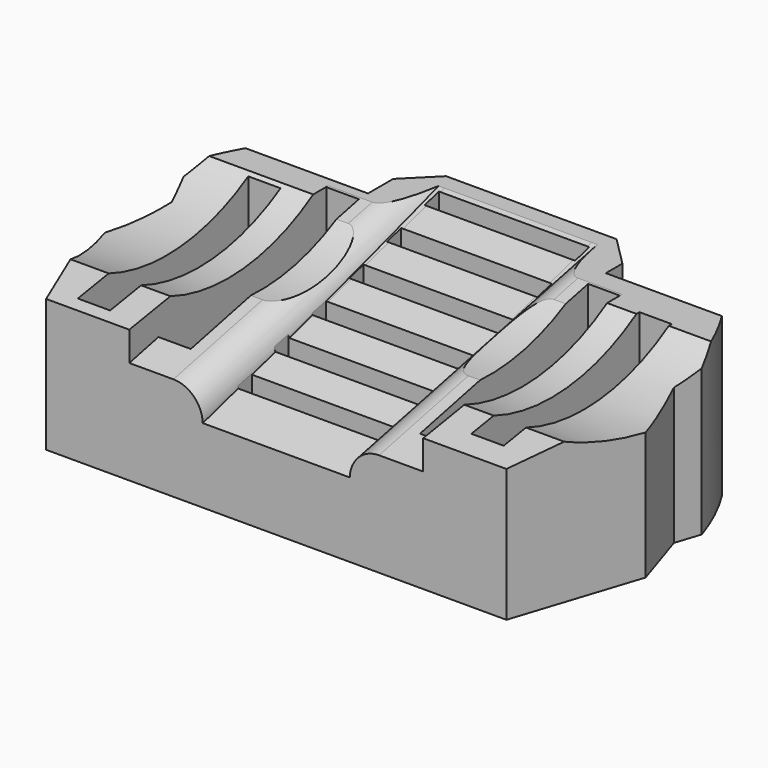
from build123d import *

# Parameters (mm, degrees)
F1_START       = 19.05
F1_DEPTH       = 31.75
F3_DEPTH       = 12.7
F5_DEPTH       = 25.4
F7_DEPTH       = 50.8
F10_T4_DEPTH   = 118.8107467306
F10_T9_DEPTH   = 118.8107467306
F11_W          = 5.588
F11_H          = 36.83
F11_H_2        = 36.322
F12_DEPTH      = 25.4
F12_DEPTH_BACK = 19.05
F13_W          = 26.0096
F13_H          = 3.048
F14_DEPTH      = 19.05
F15_W          = 26.0096
F15_H          = 3.048
F15_W_2        = 25.684906454
F16_DEPTH      = 25.4
F17_R          = 34.3708732133
F18_DEPTH      = 63.5
F19_W          = 101.6
F19_H          = 32.0445634425
F19_W_2        = 28.5529913381
F19_H_2        = 6.6054575145
F19_H_3        = 10.527446866
F19_W_3        = 20.7230086619
F19_H_4        = 8.6696632206
F19_H_5        = 7.8439861536
F20_DEPTH      = 38.1
F21_SIZE       = 5.08


# Not quite as in the source:
# - a fillet or chamfer that OpenCascade refuses, or shapes differently, is made with other operations: its cross-section is extruded or revolved along the edge and cut away or added
# - a feature of the source that left no trace in its solid (it failed there, or was rolled back) is left out


with BuildPart() as f1:
    # F0 (on Top) → F1 (new body)
    with BuildSketch(Plane.XY.offset(F1_START)):
        Polygon((-27.681270317, -38.1), (-23.1827056925, -38.1), (-29.0714032363, -33.8216107999), align=None)
        Polygon((-29.0714032363, -33.8216107999), (-23.1827056925, -38.1), (23.1827056925, -38.1), (29.0714032363, -33.8216107999), (43.3991033054, 10.2745158286), (41.1498209932, 17.1970949714), (3.6394152315, 44.45), (-3.6394152315, 44.45), (-41.1498209932, 17.1970949714), (-43.3991033054, 10.2745158286), align=None)
        with BuildLine():
            Line((23.1827056925, -38.1), (-23.1827056925, -38.1))
            Line((-23.1827056925, -38.1), (-27.681270317, -38.1))
            ThreePointArc((-27.681270317, -38.1), (0, -47.0941899427), (27.681270317, -38.1))
            Line((27.681270317, -38.1), (23.1827056925, -38.1))
        make_face()
        Polygon((-37.8114284312, -27.4716107999), (-29.0714032363, -33.8216107999), (-43.3991033054, 10.2745158286), (-46.7374958674, 0), align=None)
        Polygon((29.0714032363, -33.8216107999), (23.1827056925, -38.1), (27.681270317, -38.1), align=None)
        Polygon((-44.7892362247, 14.5529050286), (-43.3991033054, 10.2745158286), (-41.1498209932, 17.1970949714), align=None)
        Polygon((43.3991033054, 10.2745158286), (29.0714032363, -33.8216107999), (37.8114284312, -27.4716107999), (46.7374958674, 0), align=None)
        with BuildLine():
            Line((-44.7892362247, 14.5529050286), (-41.1498209932, 17.1970949714))
            Line((-41.1498209932, 17.1970949714), (-3.6394152315, 44.45))
            Line((-3.6394152315, 44.45), (0, 47.0941899427))
            ThreePointArc((0, 47.0941899427), (-27.681270317, 38.1), (-44.7892362247, 14.5529050286))
        make_face()
        Polygon((41.1498209932, 17.1970949714), (43.3991033054, 10.2745158286), (44.7892362247, 14.5529050286), align=None)
        Polygon((0, 47.0941899427), (-3.6394152315, 44.45), (3.6394152315, 44.45), align=None)
        with BuildLine():
            ThreePointArc((44.7892362247, 14.5529050286), (27.681270317, 38.1), (0, 47.0941899427))
            Line((0, 47.0941899427), (3.6394152315, 44.45))
            Line((3.6394152315, 44.45), (41.1498209932, 17.1970949714))
            Line((41.1498209932, 17.1970949714), (44.7892362247, 14.5529050286))
        make_face()
    extrude(amount=F1_DEPTH)

    # F2 (on Right) → F3 (cut, symmetric)
    with BuildSketch(Plane.YZ):
        Polygon((-44.8449260175, 25.4), (69.4550739825, 57.15), (-44.8449260175, 57.15), align=None)
    extrude(amount=F3_DEPTH, both=True, mode=Mode.SUBTRACT)

    # F4 (on Right) → F5 (cut, symmetric)
    with BuildSketch(Plane.YZ):
        Polygon((-44.8449260175, 31.75), (70.0721293688, 57.15), (-44.8449260175, 57.15), align=None)
    extrude(amount=F5_DEPTH, both=True, mode=Mode.SUBTRACT)

    # F6 (on Right) → F7 (cut, symmetric)
    with BuildSketch(Plane.YZ):
        Polygon((69.4550739825, 57.15), (-44.8449260175, 57.15), (-44.8449260175, 38.1), (5.1235620631, 46.4280813468), (48.464309937, 53.6515393258), align=None)
        Polygon((48.464309937, 46.4280813468), (48.464309937, 53.6515393258), (5.1235620631, 46.4280813468), align=None)
    extrude(amount=F7_DEPTH, both=True, mode=Mode.SUBTRACT)

    # F10: fillet of radius 5.08 on 2 edges, made by hand


with BuildPart() as f10_tool2:
    # F10_s3 → F10_t4 (new body)
    with BuildSketch(Plane(origin=(0, -48.4660281995, -10.712396973), x_dir=(1, 0, 0), z_dir=(0, 0.9764331595, 0.2158200292))):
        with BuildLine():
            ThreePointArc((-12.7, -35.6001860579), (-14.1878975516, -39.1922885063), (-17.78, -40.6801860579))
            Line((-17.78, -40.6801860579), (-12.7, -40.6801860579))
            Line((-12.7, -40.6801860579), (-12.7, -35.6001860579))
        make_face()
    extrude(amount=F10_T4_DEPTH)

    split(bisect_by=Plane(origin=(0, -9.762530517, 35.1451098613), x_dir=(1, 0, 0), z_dir=(0, -0.2676438638, 0.9635179096)), keep=Keep.TOP)


with BuildPart() as f1_1:
    add(f1.part)

    # F10_t1: cut F10_tool2
    add(f10_tool2.part, mode=Mode.SUBTRACT)


with BuildPart() as f10_tool7:
    # F10_s8 → F10_t9 (new body)
    with BuildSketch(Plane(origin=(0, -48.4660281995, -10.712396973), x_dir=(1, 0, 0), z_dir=(0, 0.9764331595, 0.2158200292))):
        with BuildLine():
            ThreePointArc((17.78, -40.6801860579), (14.1878975516, -39.1922885063), (12.7, -35.6001860579))
            Line((12.7, -35.6001860579), (12.7, -40.6801860579))
            Line((12.7, -40.6801860579), (17.78, -40.6801860579))
        make_face()
    extrude(amount=F10_T9_DEPTH)

    split(bisect_by=Plane(origin=(0, -9.762530517, 35.1451098613), x_dir=(1, 0, 0), z_dir=(0, -0.2676438638, 0.9635179096)), keep=Keep.TOP)


with BuildPart() as f1_2:
    add(f1_1.part)

    # F10_t6: cut F10_tool7
    add(f10_tool7.part, mode=Mode.SUBTRACT)

    # F11 (on offset) → F12 (cut, two sides)
    with BuildSketch(Plane.XY.offset(50.8)) as f12_sk:
        with Locations((-33.274, -0.7722239547)):
            Rectangle(F11_W, F11_H)
        with Locations((-22.606, 3.0599313468)):
            Rectangle(F11_W, F11_H_2)
        with Locations((33.274, 0.82358277)):
            Rectangle(F11_W, F11_H_2)
        with Locations((22.606, 3.0599313468)):
            Rectangle(F11_W, F11_H_2)
    extrude(amount=F12_DEPTH, mode=Mode.SUBTRACT)
    extrude(f12_sk.sketch, amount=-F12_DEPTH_BACK, mode=Mode.SUBTRACT)

    # F13 (on offset) → F14 (cut)
    with BuildSketch(Plane.XY.offset(50.8)):
        with Locations((0, 12.1964783492)):
            Rectangle(F13_W, F13_H)
        with Locations((0, 28.4524783492)):
            Rectangle(F13_W, F13_H)
        with Locations((0, 20.3244783492)):
            Rectangle(F13_W, F13_H)
    extrude(amount=-F14_DEPTH, mode=Mode.SUBTRACT)

    # F15 (on offset) → F16 (cut)
    with BuildSketch(Plane.XY.offset(50.8)):
        with Locations((0, -4.0595216508)):
            Rectangle(F15_W, F15_H)
        with Locations((0.0519962238, -12.1875216508)):
            Rectangle(F15_W_2, F15_H)
        with Locations((0, 4.0684783492)):
            Rectangle(F15_W, F15_H)
    extrude(amount=-F16_DEPTH, mode=Mode.SUBTRACT)

    # F17 (on Right) → F18 (cut, symmetric)
    with BuildSketch(Plane.YZ):
        with Locations((0, 75.4981189966)):
            Circle(F17_R)
    extrude(amount=F18_DEPTH, both=True, mode=Mode.SUBTRACT)

    # F19 (on offset) → F20 (cut, symmetric)
    with BuildSketch(Plane.XY.offset(50.8)):
        with Locations((-3.9149913381, -37.4202784151)):
            Rectangle(F19_W, F19_H)
        Polygon((46.8850086619, 51.8795326352), (-54.7149913381, 51.8795326352), (-54.7149913381, 33.7145216763), (-48.3649913381, 33.7145216763), (-48.3649913381, 40.3199791908), (-19.812, 40.3199791908), (-19.812, 33.7145216763), (19.812, 33.7145216763), (19.812, 41.5585078299), (40.5350086619, 41.5585078299), (40.5350086619, 33.7145216763), (46.8850086619, 33.7145216763), align=None)
        with Locations((-34.088495669, 37.0172504336)):
            Rectangle(F19_W_2, F19_H_2)
        with Locations((-34.088495669, 28.4507982433)):
            Rectangle(F19_W_2, F19_H_3)
        with Locations((30.173504331, 29.379690066)):
            Rectangle(F19_W_3, F19_H_4)
        with Locations((30.173504331, 37.6365147531)):
            Rectangle(F19_W_3, F19_H_5)
    extrude(amount=F20_DEPTH, both=True, mode=Mode.SUBTRACT)

    # F21
    f21_edges = [f1_2.edges().sort_by_distance(p)[0] for p in [
        (-19.812, 33.714522, 32.739041),
        (19.812, 33.714522, 32.739041),
    ]]
    chamfer(f21_edges, length=F21_SIZE)


solid = f1_2.part
